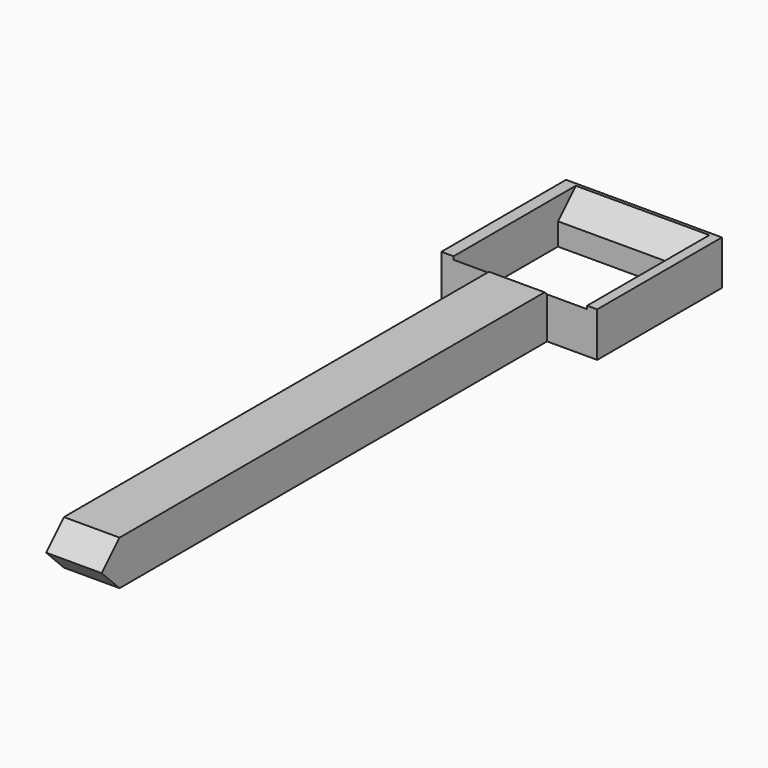
from build123d import *

# Parameters (mm, degrees)
F0_W        = 15.24
F0_H        = 12.7
F1_DEPTH    = 5.08
F2_T1_DEPTH = 15.24
F2_T3_DEPTH = 19.4141495789


# Not quite as in the source:
# - a fillet or chamfer that OpenCascade refuses, or shapes differently, is made with other operations: its cross-section is extruded or revolved along the edge and cut away or added
# - a feature names something its author has since deleted; it is built from what else it names


with BuildPart() as f1:
    # F0 (on Top) → F1 (new body)
    with BuildSketch(Plane.XY):
        Polygon((-43.6893899012, 21.153706044), (-37.9743899012, 21.153706044), (-34.7993899012, 21.153706044), (-31.6243899012, 21.153706044), (-25.9093899012, 21.153706044), (-25.9093899012, 38.933706044), (-43.6893899012, 38.933706044), align=None)
        with Locations((-34.6747071493, 29.6888263732)):
            Rectangle(F0_W, F0_H, mode=Mode.SUBTRACT)
        Polygon((-34.7993899012, 21.153706044), (-37.9743899012, 21.153706044), (-37.9743899012, -42.346293956), (-31.6243899012, -42.346293956), (-31.6243899012, 21.153706044), align=None)
    extrude(amount=F1_DEPTH)

    # F2: chamfer of 2.54 on 4 edges, made by hand

    # F2_s2 → F2_t1 (cut)
    with BuildSketch(Plane.YZ.offset(-42.2947071493)):
        Polygon((36.0388263732, 2.54), (38.5788263732, 5.08), (36.0388263732, 5.08), align=None)
        Polygon((23.3388263732, 2.54), (20.7988263732, 5.08), (23.3388263732, 5.08), align=None)
    extrude(amount=F2_T1_DEPTH, mode=Mode.SUBTRACT)

    # F2_s4 → F2_t3 (cut)
    with BuildSketch(Plane.YZ.offset(-44.5064646906)):
        Polygon((-42.346293956, 2.54), (-39.806293956, 5.08), (-42.346293956, 5.08), align=None)
        Polygon((-42.346293956, 2.54), (-39.806293956, 0), (-42.346293956, 0), align=None)
    extrude(amount=F2_T3_DEPTH, mode=Mode.SUBTRACT)


solid = f1.part
